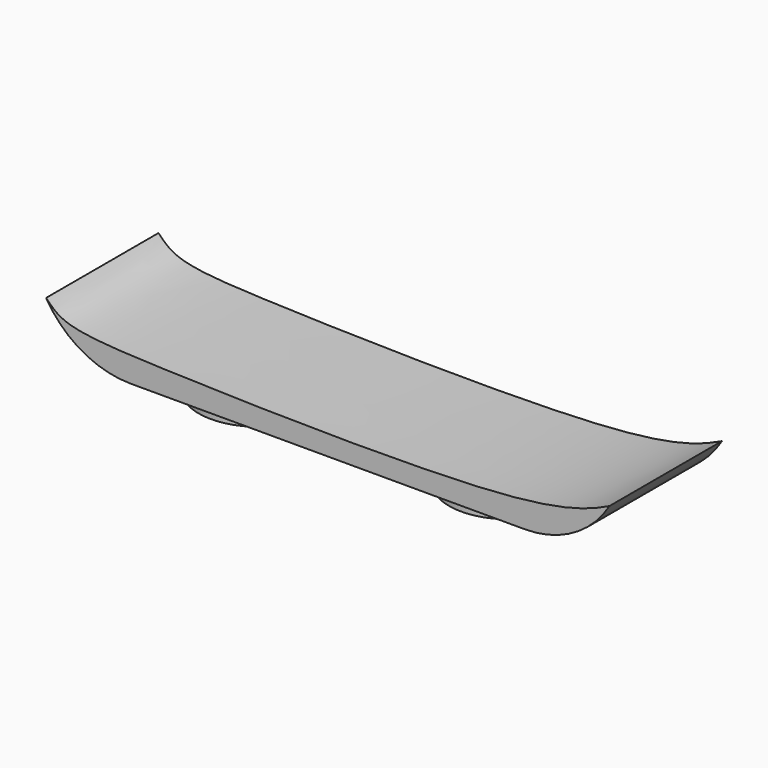
from build123d import *

# Parameters (mm, degrees)
F0_W        = 119.2497462034
F0_H        = 29.7487415373
F1_DEPTH    = 10.16
F3_DEPTH    = 35.052
F4_T1_DEPTH = 119.2514082514
F5_R        = 12.7
F6_DEPTH    = 2.54
F7_R        = 11.43
F8_DEPTH    = 0.762


# Not quite as in the source:
# - a fillet or chamfer that OpenCascade refuses, or shapes differently, is made with other operations: its cross-section is extruded or revolved along the edge and cut away or added


with BuildPart() as f1:
    # F0 (on Top) → F1 (new body)
    with BuildSketch(Plane.XY):
        Rectangle(F0_W, F0_H)
    extrude(amount=F1_DEPTH)

    # F2 (on face) → F3 (cut)
    with BuildSketch(Plane.XZ.offset(14.8743707687)):
        with BuildLine():
            Line((59.6248731017, 10.16), (-59.6248731017, 10.16))
            add(Edge.make_bspline(
                [(-59.6248731017, 10.16), (-58.6623700153, 9.1562491692), (-55.6761493356, 6.0420550119), (-35.1048833715, 4.7140763142), (36.3582789798, 3.1985096699), (54.6277439575, 7.7818062363), (58.3733948485, 9.5644064719), (59.6248731017, 10.16)],
                knots=[0, 0, 0, 0, 0.0978492049, 0.3035827346, 0.702960206, 0.9007545408, 1, 1, 1, 1], degree=3))
        make_face()
    extrude(amount=-F3_DEPTH, mode=Mode.SUBTRACT)

    # F4: fillet of radius 20.8491483247 on 2 edges, made by hand

    # F4_s2 → F4_t1 (cut)
    with BuildSketch(Plane.XZ.offset(-59.6257041257)):
        with BuildLine():
            ThreePointArc((41.7243397589, 0), (52.01577666, 2.7170411009), (59.6248731017, 10.16))
            Line((59.6248731017, 10.16), (59.6248731017, 0))
            Line((59.6248731017, 0), (41.7243397589, 0))
        make_face()
        with BuildLine():
            ThreePointArc((-41.7243397589, 0), (-52.01577666, 2.7170411009), (-59.6248731017, 10.16))
            Line((-59.6248731017, 10.16), (-59.6248731017, 0))
            Line((-59.6248731017, 0), (-41.7243397589, 0))
        make_face()
    extrude(amount=F4_T1_DEPTH, mode=Mode.SUBTRACT)

    # F5 (on face) → F6 (join)
    with BuildSketch(Plane(origin=(0, 0, 0), x_dir=(1, 0, 0), z_dir=(0, 0, -1))):
        with Locations((-26.4843397589, 0)):
            Circle(F5_R)
        with Locations((26.4843397589, 0)):
            Circle(F5_R)
    extrude(amount=F6_DEPTH)

    # F7 (on face) → F8 (cut)
    with BuildSketch(Plane(origin=(0, 0, -2.54), x_dir=(1, 0, 0), z_dir=(0, 0, -1))):
        with Locations((-26.4843397589, 0)):
            Circle(F7_R)
        with Locations((26.4843397589, 0)):
            Circle(F7_R)
    extrude(amount=-F8_DEPTH, mode=Mode.SUBTRACT)


solid = f1.part
